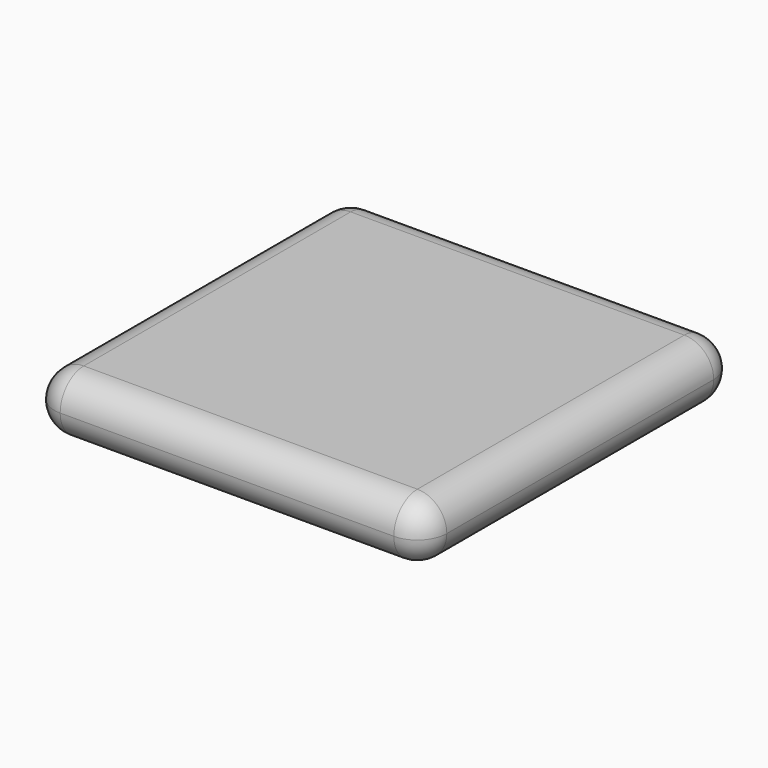
from build123d import *

# Parameters (mm, degrees)
F0_W     = 20
F0_H     = 20
F1_DEPTH = 3
F2_R     = 1.49999


# Not quite as in the source:
# - a fillet or chamfer is up to 0.001 mm smaller than in the source, because OpenCascade refuses the exact size


with BuildPart() as f1:
    # F0 (on Top) → F1 (new body)
    with BuildSketch(Plane.XY):
        with Locations((-10, 10)):
            Rectangle(F0_W, F0_H)
    extrude(amount=F1_DEPTH)

    # F2 (radius 1.5 in the source; OpenCascade refuses exactly that, so slightly less here)
    f2_edges = [f1.edges().sort_by_distance(p)[0] for p in [
        (-10, 20, 3),
        (-20, 10, 3),
        (-10, 0, 3),
        (0, 10, 3),
        (-10, 20, 0),
        (-20, 10, 0),
        (-10, 0, 0),
        (0, 10, 0),
        (-20, 0, 1.5),
        (0, 0, 1.5),
        (-20, 20, 1.5),
        (0, 20, 1.5),
    ]]
    fillet(f2_edges, radius=F2_R)


solid = f1.part
